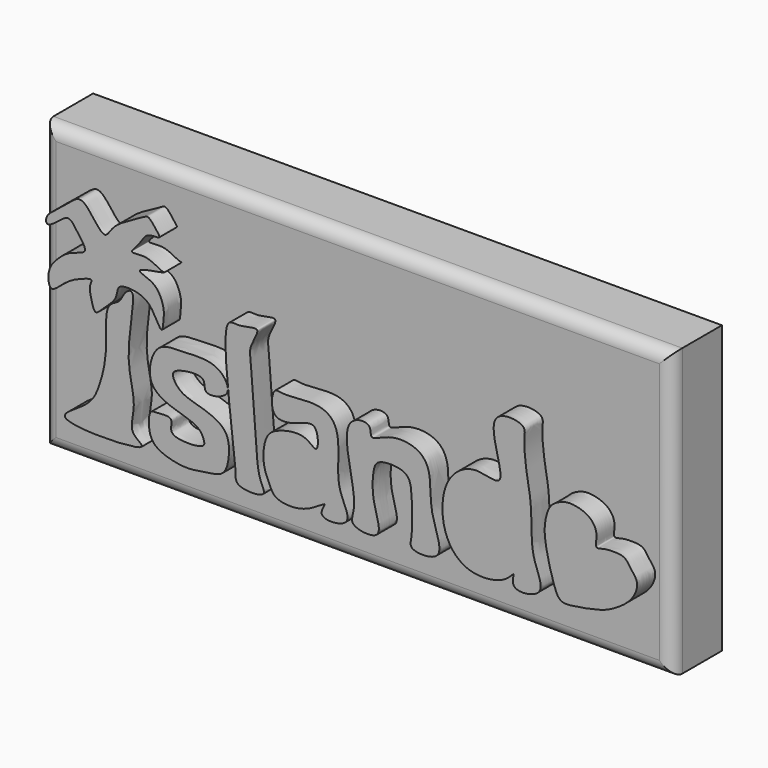
from build123d import *

# Parameters (mm, degrees)
F1_DEPTH = 11.40178
F3_DEPTH = 4.13027
F5_DEPTH = 4.1402
F6_DEPTH = 15.37349
F7_R     = 2.338141693


# Not quite as in the source:
# - a feature of the source that left no trace in its solid (it failed there, or was rolled back) is left out


with BuildPart() as f1:
    # F0 (on Front) → F1 (new body)
    with BuildSketch(Plane.XZ):
        Polygon((56.4285255969, 42.183291167), (-58.6567521095, 42.0997776091), (-58.6567521095, -10.2648623288), (56.4285255969, -10.2648623288), align=None)
    extrude(amount=F1_DEPTH)

    # F2 (on face) → F3 (join)
    with BuildSketch(Plane.XZ.offset(11.40178)):
        with BuildLine():
            add(Edge.make_bspline(
                [(-43.3281445523, 19.1339574578), (-44.1515090731, 17.7944839027), (-43.3947714278, 11.4987350744), (-45.0856873065, 5.4825404345), (-46.7725247024, 1.7619730372), (-56.6178752304, -2.8775529377), (-33.7771540298, -2.4275794149), (-40.0592444338, -0.0712260113), (-37.8943868514, 5.0547699232), (-40.9321381761, 11.7125197131), (-37.8920425362, 23.9198647824), (-40.6542449146, 22.3163999481), (-41.2219501742, 20.182210178), (-42.8692491746, 19.8805019197), (-43.3281445523, 19.1339574578)],
                knots=[0, 0, 0, 0, 0.1001433158, 0.1940002234, 0.2734970297, 0.3537986525, 0.491789473, 0.5458632605, 0.6241168685, 0.7304389957, 0.8481545423, 0.8900207729, 0.9441859546, 1, 1, 1, 1], degree=3))
        make_face()
        with BuildLine():
            add(Edge.make_bspline(
                [(-26.1220727116, 12.9132140428), (-25.6809252913, 12.4353380204), (-26.4642096222, 10.2055116326), (-20.4917173497, 11.4791026779), (-22.480115742, 15.4344376324), (-25.7397994944, 16.4546727718), (-30.039604588, 16.1567733931), (-34.1169561087, 16.1875975666), (-35.9273792518, 12.8755064943), (-36.0274470516, 8.1855783022), (-30.6637639327, 6.1101741319), (-26.781734654, 5.202300805), (-25.8441728417, 3.0986102963), (-25.8469614184, 1.8461006638), (-30.0550482435, 1.5782292064), (-32.4334773314, 2.4554307969), (-31.2924638616, 5.2477360702), (-34.5744349461, 4.7184158365), (-36.0579499386, 4.9245836886), (-36.1378358483, 1.2438029545), (-34.7635581495, -1.3008242192), (-29.1941154878, -2.6523132694), (-25.8187285052, -1.7875161271), (-22.1883249913, -1.5819851887), (-21.2193147286, 1.8655766547), (-21.3515888369, 6.5276285567), (-26.5374995492, 8.4445307075), (-30.3720746075, 9.2644105467), (-32.0544640906, 12.0098832182), (-30.6623347223, 13.1605514347), (-26.7938641855, 13.6409368462), (-26.1220727116, 12.9132140428)],
                knots=[0, 0, 0, 0, 0.0268930206, 0.0649913539, 0.0988544107, 0.1346503362, 0.1756037706, 0.213403019, 0.249023428, 0.2881682481, 0.3330472229, 0.3720581313, 0.3994771141, 0.4172063961, 0.4558637815, 0.4844718947, 0.510685989, 0.5416050751, 0.5633189243, 0.5971726226, 0.63001784, 0.6749168867, 0.712580885, 0.7469828474, 0.7815706573, 0.8213882982, 0.8650971, 0.9045590075, 0.9352419033, 0.9590465656, 1, 1, 1, 1], degree=3))
        make_face()
        with BuildLine():
            add(Edge.make_bspline(
                [(-21.6268710792, 23.2022311538), (-22.8629697708, 20.396395146), (-19.8658383261, 0.7578510741), (-20.2640035323, -0.8966101309), (-19.6471519735, -2.5327714924), (-14.0050556046, -2.5848648709), (-15.9524937856, 0.2525017099), (-16.3844908975, 4.9347872506), (-16.7702005794, 11.8012109793), (-17.4138117975, 18.7897248591), (-17.6882643671, 21.1341945173), (-14.9888121465, 25.1145100072), (-19.5743042819, 23.3266944932), (-21.231097804, 24.1006019022), (-21.6268710792, 23.2022311538)],
                knots=[0, 0, 0, 0, 0.1895009406, 0.2477594711, 0.2932284202, 0.3755834512, 0.4325921275, 0.520567841, 0.6292538239, 0.7342323419, 0.7991153824, 0.8672931209, 0.9393257121, 1, 1, 1, 1], degree=3))
        make_face()
        with BuildLine():
            add(Edge.make_bspline(
                [(-5.3442530334, 8.5179060698), (-5.6909922811, 8.2076675513), (-7.3958149108, 10.4068781927), (-12.2834910141, 9.4047076068), (-14.902752841, 7.79502382), (-15.3225793617, 2.6068665688), (-13.8792963536, 0.0955183947), (-13.1768530404, -2.2613688974), (-7.4285950207, -2.7617795211), (-2.7150872901, 1.2456319366), (-5.8439100927, -2.7422374554), (2.0894556486, -2.351207913), (-1.5925237585, 3.0021931577), (-1.3017910922, 8.0408005371), (-1.2936740794, 13.6168013212), (-4.9396269758, 16.251420056), (-11.3850881216, 15.0087232542), (-13.3949145261, 16.0584953708), (-14.0168362415, 10.2504125951), (-8.7084206824, 11.2951361548), (-5.0960960914, 13.1470414038), (-4.9221570676, 8.8955686157), (-5.3442530334, 8.5179060698)],
                knots=[0, 0, 0, 0, 0.0388618845, 0.0958553914, 0.140269278, 0.1967697692, 0.2410614646, 0.2778352741, 0.3393402282, 0.3902307479, 0.425503914, 0.4797356168, 0.5341454019, 0.5952194069, 0.6541117697, 0.7053249544, 0.7710752876, 0.8029398913, 0.8529298001, 0.9068280119, 0.9526922759, 1, 1, 1, 1], degree=3))
        make_face()
        with BuildLine():
            add(Edge.make_bspline(
                [(0.7492440636, 14.5115079358), (-0.854221182, 11.9905762629), (2.9187519947, 1.8594345853), (-0.0410029969, -1.8790029496), (7.4652542075, -2.8706996682), (4.6915882761, 3.2065686591), (4.932387856, 8.4314526014), (5.8615471371, 10.5976017744), (11.4735173077, 10.5217809544), (12.1955321798, 7.0149347231), (12.3268783392, 0.1849072738), (11.3443327376, -2.4050017632), (18.9631688245, -2.5160609468), (15.1245076582, 4.888256769), (15.8316429622, 10.7977310388), (13.8687471359, 14.757603842), (8.2494090922, 15.4556776093), (4.1742085503, 12.7070767738), (4.9833400876, 16.1140057217), (1.6009524619, 15.8505445524), (0.7492440636, 14.5115079358)],
                knots=[0, 0, 0, 0, 0.0945559803, 0.1427190092, 0.197110927, 0.2552849624, 0.317454036, 0.3543894091, 0.4106465584, 0.457900445, 0.5281659426, 0.5645454775, 0.6208856141, 0.6866322658, 0.7533141427, 0.8044493101, 0.8662347626, 0.9154560161, 0.9497749498, 1, 1, 1, 1], degree=3))
        make_face()
        with BuildLine():
            add(Edge.make_bspline(
                [(28.2199196517, 14.5115079358), (27.7604857244, 13.5387092432), (23.5359022403, 15.5358777127), (18.7487737533, 12.3447277553), (17.35927978, 7.1347864952), (18.1766806213, 1.3649136106), (22.385080362, -2.910865627), (29.2006680445, -2.0594771109), (31.1797002925, 0.9401240614), (29.7054593879, -3.0222502134), (37.4304351492, -2.0181803887), (33.5850899736, 3.9616567552), (34.2674709096, 11.7889142665), (33.0205143362, 16.904019689), (32.5088184788, 22.5504106341), (33.1634797138, 25.0031681962), (24.1808974973, 25.8845538968), (28.9084861213, 15.9694685292), (28.2199196517, 14.5115079358)],
                knots=[0, 0, 0, 0, 0.0582267191, 0.1237804682, 0.1882857817, 0.2554611562, 0.3218266618, 0.3945354059, 0.4329327835, 0.4718440775, 0.5322996028, 0.5968534133, 0.6773266805, 0.7443077585, 0.811027092, 0.8496075465, 0.9127339884, 1, 1, 1, 1], degree=3))
        make_face()
        with BuildLine():
            add(Edge.make_bspline(
                [(45.9010452032, 9.3170534819), (45.6787030959, 9.5567407169), (46.1476392458, 11.2851085319), (45.3595509893, 13.2490178572), (43.5815194199, 14.4491058501), (41.0885664585, 14.9551374857), (39.4998676047, 14.5713302253), (37.256908791, 13.5491641501), (36.3504363041, 10.254463245), (36.424794843, 7.4834688282), (37.1473037766, 3.9482580049), (38.2693039305, 0.0689540415), (39.3242705661, -1.8641318125), (42.3111594321, -1.492186718), (45.8190941995, -0.8262796763), (48.1108523755, -0.1054394769), (50.8955673683, 1.5295486439), (52.9523789811, 3.5994080436), (53.6374290193, 6.2127437495), (52.3207963807, 7.5518891047), (51.2914833701, 9.533265848), (49.0663589804, 9.6588313465), (47.1438164107, 9.5433708496), (46.0752163043, 9.129295121), (45.9010452032, 9.3170534819)],
                knots=[0, 0, 0, 0, 0.0392539018, 0.0818439662, 0.1240493999, 0.1698599185, 0.2071899394, 0.251050007, 0.3033501762, 0.3523084001, 0.4083392524, 0.4676276132, 0.507298086, 0.5553741092, 0.6114049508, 0.656980284, 0.7089274477, 0.7593772881, 0.8042646427, 0.8429616052, 0.8849707516, 0.9267557295, 0.96925056, 1, 1, 1, 1], degree=3))
        make_face()
    extrude(amount=F3_DEPTH)

    # F4 (on Front) → F5 (join)
    with BuildSketch(Plane.XZ):
        with BuildLine():
            add(Edge.make_bspline(
                [(-39.9339720607, 23.1057163328), (-40.7047807459, 23.1128160438), (-42.0460945661, 22.846255951), (-41.803841963, 20.5508526331), (-44.5534194717, 18.3906232293), (-46.070972153, 16.6095960648), (-46.703875452, 19.2466356909), (-47.1823581071, 21.1310383451), (-46.1159221818, 22.685653285), (-49.5599934164, 21.4607730961), (-51.5505588792, 20.2286981538), (-53.4988277623, 18.3168907257), (-54.4974336798, 18.4948678811), (-54.7392376116, 21.5220960647), (-52.8337947425, 23.7136049684), (-50.63822408, 25.5589536413), (-46.937426151, 26.1362838431), (-49.0497268126, 28.7599197048), (-50.2234695237, 30.6304946557), (-51.4027687002, 30.9235565296), (-53.4111368967, 29.0719986746), (-54.9462464421, 28.2475139905), (-55.0882258025, 30.0357655845), (-52.7669278951, 31.555353421), (-50.3692689298, 33.7596753729), (-48.6243300101, 34.8980155186), (-46.7000968835, 33.0336483591), (-44.2327705078, 29.2482984556), (-42.9115052132, 32.0387146609), (-40.3224708883, 33.7654204769), (-37.0569826007, 35.4733666596), (-36.1596155008, 35.9708304323), (-34.7035219365, 34.0149429299), (-33.7651288224, 32.7921577587), (-36.7461021963, 33.2372206875), (-37.6063170082, 30.8852142055), (-40.2618516013, 28.6286301337), (-36.5001515815, 29.5958185946), (-34.0922730898, 27.826359563), (-32.7961958724, 27.7145382887), (-36.1390391475, 27.2925582883), (-38.7574571359, 26.4917358377), (-35.3919968111, 25.6566119121), (-34.0008975937, 23.9340467528), (-33.2750054729, 21.4752093979), (-33.5111914094, 20.0070291747), (-33.6376801265, 17.4112035773), (-35.1898970443, 20.5590049625), (-36.6262499842, 22.6098922446), (-38.9245408774, 23.0964187342), (-39.9339720607, 23.1057163328)],
                knots=[0, 0, 0, 0, 0.0191620851, 0.0383241673, 0.0652369205, 0.0830641079, 0.1029913541, 0.1240929616, 0.1378376133, 0.1606939823, 0.1849703886, 0.2073531607, 0.2185756069, 0.2413829806, 0.2655609664, 0.2903469063, 0.313579697, 0.3357568209, 0.3573788204, 0.3710097754, 0.394659052, 0.4108140437, 0.4254552575, 0.4489261654, 0.4752739106, 0.4935758411, 0.5161688521, 0.5430696306, 0.5627872411, 0.589179509, 0.6162229367, 0.6287030879, 0.6505129884, 0.6640976229, 0.6841417449, 0.7071671677, 0.7277737396, 0.7498864348, 0.7755375015, 0.785365721, 0.8093474182, 0.8284008333, 0.8497942429, 0.8718419348, 0.893713409, 0.9124646289, 0.9296851439, 0.9511732104, 0.9749058274, 1, 1, 1, 1], degree=3))
        make_face()
    extrude(amount=F5_DEPTH)

    # F4 (on Front) → F6 (join)
    with BuildSketch(Plane.XZ):
        with BuildLine():
            add(Edge.make_bspline(
                [(-39.9339720607, 23.1057163328), (-40.7047807459, 23.1128160438), (-42.0460945661, 22.846255951), (-41.803841963, 20.5508526331), (-44.5534194717, 18.3906232293), (-46.070972153, 16.6095960648), (-46.703875452, 19.2466356909), (-47.1823581071, 21.1310383451), (-46.1159221818, 22.685653285), (-49.5599934164, 21.4607730961), (-51.5505588792, 20.2286981538), (-53.4988277623, 18.3168907257), (-54.4974336798, 18.4948678811), (-54.7392376116, 21.5220960647), (-52.8337947425, 23.7136049684), (-50.63822408, 25.5589536413), (-46.937426151, 26.1362838431), (-49.0497268126, 28.7599197048), (-50.2234695237, 30.6304946557), (-51.4027687002, 30.9235565296), (-53.4111368967, 29.0719986746), (-54.9462464421, 28.2475139905), (-55.0882258025, 30.0357655845), (-52.7669278951, 31.555353421), (-50.3692689298, 33.7596753729), (-48.6243300101, 34.8980155186), (-46.7000968835, 33.0336483591), (-44.2327705078, 29.2482984556), (-42.9115052132, 32.0387146609), (-40.3224708883, 33.7654204769), (-37.0569826007, 35.4733666596), (-36.1596155008, 35.9708304323), (-34.7035219365, 34.0149429299), (-33.7651288224, 32.7921577587), (-36.7461021963, 33.2372206875), (-37.6063170082, 30.8852142055), (-40.2618516013, 28.6286301337), (-36.5001515815, 29.5958185946), (-34.0922730898, 27.826359563), (-32.7961958724, 27.7145382887), (-36.1390391475, 27.2925582883), (-38.7574571359, 26.4917358377), (-35.3919968111, 25.6566119121), (-34.0008975937, 23.9340467528), (-33.2750054729, 21.4752093979), (-33.5111914094, 20.0070291747), (-33.6376801265, 17.4112035773), (-35.1898970443, 20.5590049625), (-36.6262499842, 22.6098922446), (-38.9245408774, 23.0964187342), (-39.9339720607, 23.1057163328)],
                knots=[0, 0, 0, 0, 0.0191620851, 0.0383241673, 0.0652369205, 0.0830641079, 0.1029913541, 0.1240929616, 0.1378376133, 0.1606939823, 0.1849703886, 0.2073531607, 0.2185756069, 0.2413829806, 0.2655609664, 0.2903469063, 0.313579697, 0.3357568209, 0.3573788204, 0.3710097754, 0.394659052, 0.4108140437, 0.4254552575, 0.4489261654, 0.4752739106, 0.4935758411, 0.5161688521, 0.5430696306, 0.5627872411, 0.589179509, 0.6162229367, 0.6287030879, 0.6505129884, 0.6640976229, 0.6841417449, 0.7071671677, 0.7277737396, 0.7498864348, 0.7755375015, 0.785365721, 0.8093474182, 0.8284008333, 0.8497942429, 0.8718419348, 0.893713409, 0.9124646289, 0.9296851439, 0.9511732104, 0.9749058274, 1, 1, 1, 1], degree=3))
        make_face()
    extrude(amount=F6_DEPTH)

    # F7
    f7_edges = [f1.edges().sort_by_distance(p)[0] for p in [
        (-58.656752, -11.40178, 15.917458),
        (-1.114113, -11.40178, 42.141534),
        (56.428526, -11.40178, 15.959214),
        (-1.114113, -11.40178, -10.264862),
    ]]
    fillet(f7_edges, radius=F7_R)


solid = f1.part
